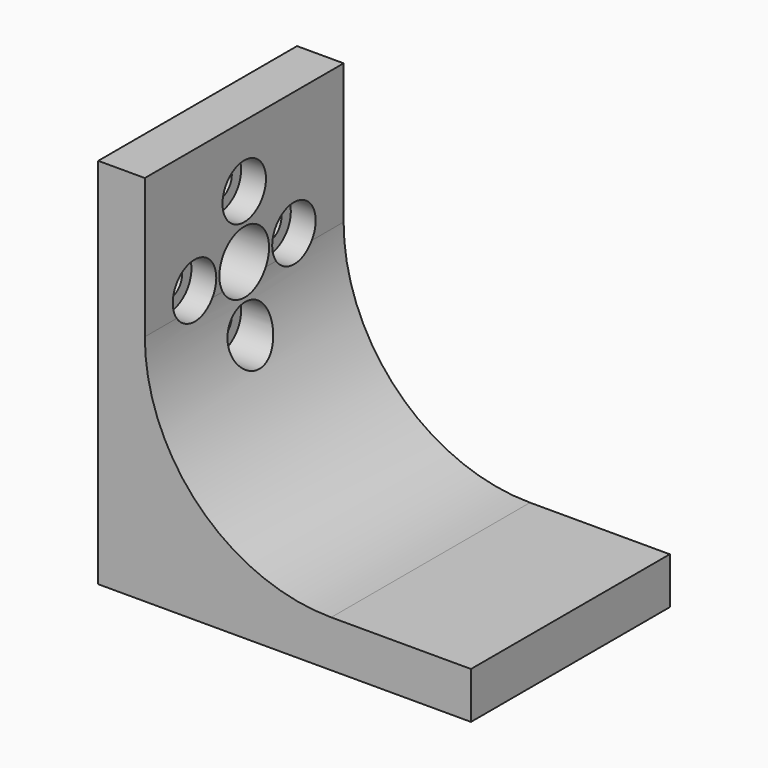
from build123d import *

# Parameters (mm, degrees)
F5_DEPTH      = 16
F7_R          = 24
F6_R          = 2
F6_R_2        = 4
F8_DEPTH      = 6.001
F8_DEPTH_BACK = 42.001
F6_R_3        = 3.5
F9_DEPTH      = 3.2
F9_DEPTH_BACK = 42.001


with BuildPart() as f5:
    # F4 (on Front) → F5 (new body, symmetric)
    with BuildSketch(Plane.XZ):
        Polygon((6, 48), (0, 48), (0, 0), (48, 0), (48, 6), (6, 6), align=None)
    extrude(amount=F5_DEPTH, both=True)

    # F7
    f7_edges = [f5.edges().sort_by_distance(p)[0] for p in [
        (6, 0, 6),
    ]]
    fillet(f7_edges, radius=F7_R)

    # F6 (on face) → F8 (cut, two sides)
    with BuildSketch(Plane.YZ.offset(6)) as f8_sk:
        with Locations((-8, 32)):
            Circle(F6_R)
        with Locations((0, 40)):
            Circle(F6_R)
        with Locations((8, 32)):
            Circle(F6_R)
        with Locations((0, 32)):
            Circle(F6_R_2)
        with Locations((0, 24)):
            Circle(F6_R)
    extrude(amount=-F8_DEPTH, mode=Mode.SUBTRACT)
    extrude(f8_sk.sketch, amount=F8_DEPTH_BACK, mode=Mode.SUBTRACT)

    # F6 (on face) → F9 (cut, two sides)
    with BuildSketch(Plane.YZ.offset(6)) as f9_sk:
        with Locations((-8, 32)):
            Circle(F6_R_3)
        with Locations((-8, 32)):
            Circle(F6_R, mode=Mode.SUBTRACT)
        with Locations((0, 40)):
            Circle(F6_R_3)
        with Locations((0, 40)):
            Circle(F6_R, mode=Mode.SUBTRACT)
        with Locations((8, 32)):
            Circle(F6_R_3)
        with Locations((8, 32)):
            Circle(F6_R, mode=Mode.SUBTRACT)
        with Locations((0, 24)):
            Circle(F6_R_3)
        with Locations((0, 24)):
            Circle(F6_R, mode=Mode.SUBTRACT)
    extrude(amount=-F9_DEPTH, mode=Mode.SUBTRACT)
    extrude(f9_sk.sketch, amount=F9_DEPTH_BACK, mode=Mode.SUBTRACT)


solid = f5.part
